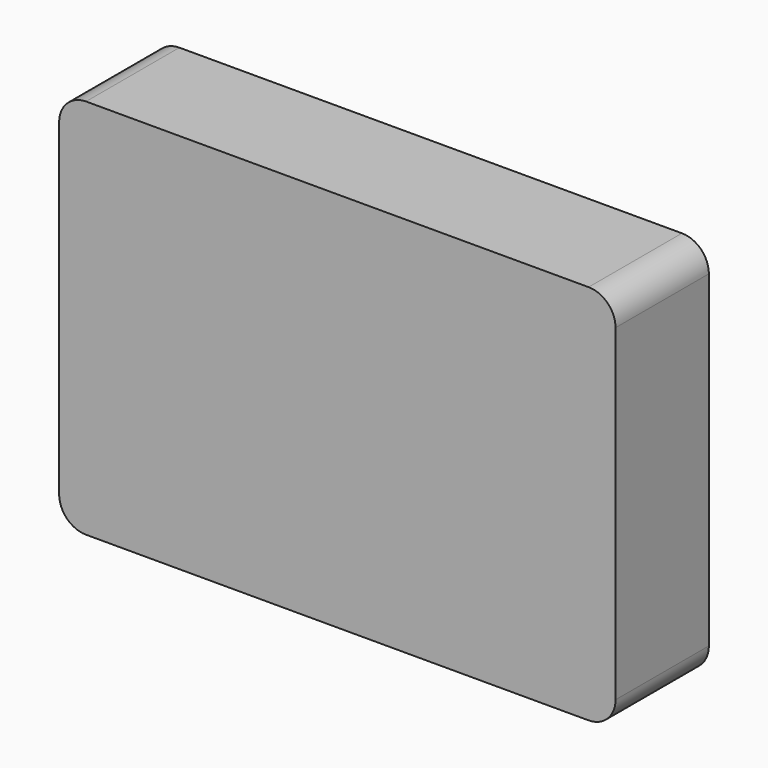
from build123d import *

# Parameters (mm, degrees)
F1_DEPTH = 7.9375
F3_DEPTH = 4.7625
F5_DEPTH = 6.35


# Not quite as in the source:
# - a pattern or mirror of a feature is missing from the dataset's text; its kind, count and spacing are read off the source's solid


with BuildPart() as f1:
    # F0 (on Front) → F1 (new body, symmetric)
    with BuildSketch(Plane.XZ):
        with BuildLine():
            Line((44.45, 33.734375), (-44.45, 33.734375))
            ThreePointArc((-44.45, 33.734375), (-47.8175960454, 32.3394710454), (-49.2125, 28.971875))
            Line((-49.2125, 28.971875), (-49.2125, -28.971875))
            ThreePointArc((-49.2125, -28.971875), (-47.8175960454, -32.3394710454), (-44.45, -33.734375))
            Line((-44.45, -33.734375), (44.45, -33.734375))
            ThreePointArc((44.45, -33.734375), (47.8175960454, -32.3394710454), (49.2125, -28.971875))
            Line((49.2125, -28.971875), (49.2125, 28.971875))
            ThreePointArc((49.2125, 28.971875), (47.8175960454, 32.3394710454), (44.45, 33.734375))
        make_face()
        with BuildLine():
            ThreePointArc((-42.8625, 27.384375), (-42.3975320151, 28.5069070151), (-41.275, 28.971875))
            Line((-41.275, 28.971875), (41.275, 28.971875))
            ThreePointArc((41.275, 28.971875), (42.3975320151, 28.5069070151), (42.8625, 27.384375))
            Line((42.8625, 27.384375), (42.8625, -27.384375))
            ThreePointArc((42.8625, -27.384375), (42.3975320151, -28.5069070151), (41.275, -28.971875))
            Line((41.275, -28.971875), (-41.275, -28.971875))
            ThreePointArc((-41.275, -28.971875), (-42.3975320151, -28.5069070151), (-42.8625, -27.384375))
            Line((-42.8625, -27.384375), (-42.8625, 27.384375))
        make_face(mode=Mode.SUBTRACT)
    extrude(amount=F1_DEPTH, both=True)

    # F2 (on face) → F3 (join)
    with BuildSketch(Plane.XZ.offset(7.9375)):
        with BuildLine():
            Line((-49.2125, 28.971875), (-49.2125, -28.971875))
            ThreePointArc((-49.2125, -28.971875), (-47.8175960454, -32.3394710454), (-44.45, -33.734375))
            Line((-44.45, -33.734375), (44.45, -33.734375))
            ThreePointArc((44.45, -33.734375), (47.8175960454, -32.3394710454), (49.2125, -28.971875))
            Line((49.2125, -28.971875), (49.2125, 28.971875))
            ThreePointArc((49.2125, 28.971875), (47.8175960454, 32.3394710454), (44.45, 33.734375))
            Line((44.45, 33.734375), (-44.45, 33.734375))
            ThreePointArc((-44.45, 33.734375), (-47.8175960454, 32.3394710454), (-49.2125, 28.971875))
        make_face()
        with BuildLine():
            Line((41.275, -28.971875), (-41.275, -28.971875))
            ThreePointArc((-41.275, -28.971875), (-42.3975320151, -28.5069070151), (-42.8625, -27.384375))
            Line((-42.8625, -27.384375), (-42.8625, 27.384375))
            ThreePointArc((-42.8625, 27.384375), (-42.3975320151, 28.5069070151), (-41.275, 28.971875))
            Line((-41.275, 28.971875), (41.275, 28.971875))
            ThreePointArc((41.275, 28.971875), (42.3975320151, 28.5069070151), (42.8625, 27.384375))
            Line((42.8625, 27.384375), (42.8625, -27.384375))
            ThreePointArc((42.8625, -27.384375), (42.3975320151, -28.5069070151), (41.275, -28.971875))
        make_face(mode=Mode.SUBTRACT)
        with BuildLine():
            ThreePointArc((-42.8625, -27.384375), (-42.3975320151, -28.5069070151), (-41.275, -28.971875))
            Line((-41.275, -28.971875), (41.275, -28.971875))
            ThreePointArc((41.275, -28.971875), (42.3975320151, -28.5069070151), (42.8625, -27.384375))
            Line((42.8625, -27.384375), (42.8625, 27.384375))
            ThreePointArc((42.8625, 27.384375), (42.3975320151, 28.5069070151), (41.275, 28.971875))
            Line((41.275, 28.971875), (-41.275, 28.971875))
            ThreePointArc((-41.275, 28.971875), (-42.3975320151, 28.5069070151), (-42.8625, 27.384375))
            Line((-42.8625, 27.384375), (-42.8625, -27.384375))
        make_face()
    extrude(amount=F3_DEPTH)

    # F4 (on Top) → F5 (cut, symmetric)
    with BuildSketch(Plane.XY):
        with BuildLine():
            Line((-43.9211182963, -1.5875), (-42.8625, -1.5875))
            Line((-42.8625, -1.5875), (-42.8625, 1.5875))
            Line((-42.8625, 1.5875), (-42.8625, 7.9375))
            Line((-42.8625, 7.9375), (-45.6565, 7.9375))
            Line((-45.6565, 7.9375), (-45.6565, 4.8221398621))
            ThreePointArc((-45.6565, 4.8221398621), (-45.712945133, 4.3067430314), (-45.8796045821, 3.8157801263))
            Line((-45.8796045821, 3.8157801263), (-46.4493954179, 2.5938597358))
            ThreePointArc((-46.4493954179, 2.5938597358), (-46.6725, 1.5875), (-46.4493954179, 0.5811402642))
            Line((-46.4493954179, 0.5811402642), (-46.0792637142, -0.2126097358))
            ThreePointArc((-46.0792637142, -0.2126097358), (-45.2005629887, -1.2145758803), (-43.9211182963, -1.5875))
        make_face()
    f5 = extrude(amount=F5_DEPTH, both=True, mode=Mode.SUBTRACT)

    # F5_copies: F5 across plane
    add(f5.mirror(Plane(origin=(0, 0, 0), x_dir=(0, 0, 1), z_dir=(1, 0, 0))), mode=Mode.SUBTRACT)


solid = f1.part
